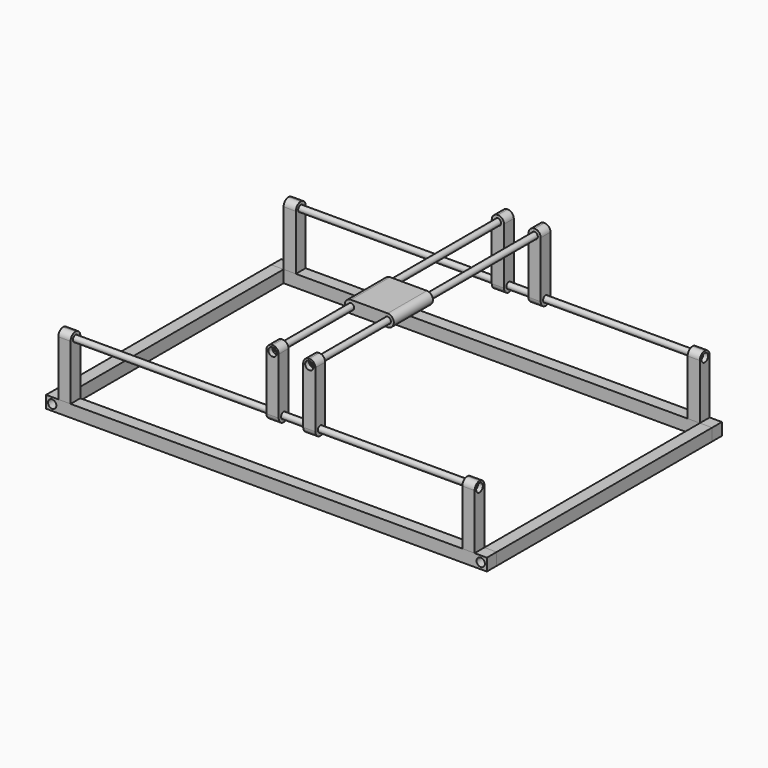
from build123d import *

# Parameters (mm, degrees)
F0_R                   = 2.159
F1_DEPTH               = 6.35
F0_W                   = 6.35
F0_H                   = 139.7
F2_DEPTH               = 6.35
F5_D                   = 2.54
F5_DEPTH               = 14.2875
F5_CBORE_D             = 4.318
F5_CBORE_DEPTH         = 6.35
F5_TIP                 = 0.7630929862
F5_2_D                 = 2.54
F5_2_DEPTH             = 14.2875
F5_2_CBORE_D           = 4.318
F5_2_CBORE_DEPTH       = 6.35
F5_2_TIP               = 0.7630929862
F5_3_D                 = 2.54
F5_3_DEPTH             = 14.2875
F5_3_CBORE_D           = 4.318
F5_3_CBORE_DEPTH       = 6.35
F5_3_TIP               = 0.7630929862
F5_ON_F3_D             = 2.54
F5_ON_F3_DEPTH         = 14.2875
F5_ON_F3_CBORE_D       = 4.318
F5_ON_F3_CBORE_DEPTH   = 6.35
F5_ON_F3_TIP           = 0.7630929862
F5_ON_F3_2_D           = 2.54
F5_ON_F3_2_DEPTH       = 14.2875
F5_ON_F3_2_CBORE_D     = 4.318
F5_ON_F3_2_CBORE_DEPTH = 6.35
F5_ON_F3_2_TIP         = 0.7630929862
F5_ON_F3_3_D           = 2.54
F5_ON_F3_3_DEPTH       = 14.2875
F5_ON_F3_3_CBORE_D     = 4.318
F5_ON_F3_3_CBORE_DEPTH = 6.35
F5_ON_F3_3_TIP         = 0.7630929862
F6_W                   = 6.35
F6_H                   = 6.35
F7_DEPTH               = 31.75
F8_R                   = 3.17499
F9_D                   = 2.5146
F9_DEPTH               = 15.2146
F9_CBORE_D             = 4.318
F9_CBORE_DEPTH         = 2.5146
F9_TIP                 = 0.7554620563
F9_2_D                 = 2.5146
F9_2_DEPTH             = 15.2146
F9_2_CBORE_D           = 4.318
F9_2_CBORE_DEPTH       = 2.5146
F9_2_TIP               = 0.7554620563
F9_3_D                 = 2.5146
F9_3_DEPTH             = 15.2146
F9_3_CBORE_D           = 4.318
F9_3_CBORE_DEPTH       = 2.5146
F9_3_TIP               = 0.7554620563
F10_R                  = 1.651
F11_DEPTH              = 1.27
F13_D                  = 2.5146
F13_CBORE_D            = 4.318
F13_CBORE_DEPTH        = 2.5146
F14_R                  = 1.5875
F15_DEPTH              = 102.87
F19_DEPTH              = 6.35
F21_DEPTH              = 6.35
F22_D                  = 2.5146
F22_CBORE_D            = 4.318
F22_CBORE_DEPTH        = 2.5146
F23_R                  = 1.6891
F23_R_2                = 1.2573
F24_DEPTH              = 1.27
F28_R                  = 1.5875
F29_DEPTH              = 71.12
F30_R                  = 1.651
F31_DEPTH              = 25.4


# Not quite as in the source:
# - a fillet or chamfer is up to 0.001 mm smaller than in the source, because OpenCascade refuses the exact size


with BuildPart() as f1:
    # F0 (on Top) → F1 (new body)
    with BuildSketch(Plane.XY):
        Polygon((-107.95, 69.85), (107.95, 69.85), (114.3, 69.85), (114.3, 76.2), (-114.3, 76.2), (-114.3, 69.85), align=None)
        with Locations((-104.775, 73.025)):
            Circle(F0_R, mode=Mode.SUBTRACT)
        with Locations((104.775, 73.025)):
            Circle(F0_R, mode=Mode.SUBTRACT)
        with Locations((-104.775, 73.025)):
            Circle(F0_R)
        with Locations((104.775, 73.025)):
            Circle(F0_R)
    extrude(amount=F1_DEPTH)

    # F5 on F3
    with Locations(Plane(origin=(0, 76.2, 0), x_dir=(-1, 0, 0), z_dir=(0, 1, 0))):
        with Locations((111.125, 3.175), (-111.125, 3.175)):
            CounterBoreHole(F5_ON_F3_D / 2, F5_ON_F3_CBORE_D / 2, F5_ON_F3_CBORE_DEPTH, depth=F5_ON_F3_DEPTH)
            with Locations((0, 0, -(F5_ON_F3_DEPTH + F5_ON_F3_TIP / 2))):  # 118° drill point
                Cone(0, F5_ON_F3_D / 2, F5_ON_F3_TIP, mode=Mode.SUBTRACT)

    # F9
    with Locations(Plane(origin=(0, 0, 0), x_dir=(1, 0, 0), z_dir=(0, 0, -1))):
        with Locations((-104.775, 73.025), (104.775, 73.025), (104.775, -73.025), (-104.775, -73.025)):
            CounterBoreHole(F9_D / 2, F9_CBORE_D / 2, F9_CBORE_DEPTH, depth=F9_DEPTH)
            with Locations((0, 0, -(F9_DEPTH + F9_TIP / 2))):  # 118° drill point
                Cone(0, F9_D / 2, F9_TIP, mode=Mode.SUBTRACT)


with BuildPart() as f1b:
    # F0 (on Top) → F1, piece 2 (new body)
    with BuildSketch(Plane.XY):
        Polygon((114.3, -69.85), (107.95, -69.85), (-107.95, -69.85), (-114.3, -69.85), (-114.3, -76.2), (114.3, -76.2), align=None)
        with Locations((-104.775, -73.025)):
            Circle(F0_R, mode=Mode.SUBTRACT)
        with Locations((104.775, -73.025)):
            Circle(F0_R, mode=Mode.SUBTRACT)
        with Locations((104.775, -73.025)):
            Circle(F0_R)
        with Locations((-104.775, -73.025)):
            Circle(F0_R)
    extrude(amount=F1_DEPTH)

    # F5
    with Locations(Plane.XZ.offset(76.2)):
        with Locations((111.125, 3.175), (-111.125, 3.175)):
            CounterBoreHole(F5_D / 2, F5_CBORE_D / 2, F5_CBORE_DEPTH, depth=F5_DEPTH)
            with Locations((0, 0, -(F5_DEPTH + F5_TIP / 2))):  # 118° drill point
                Cone(0, F5_D / 2, F5_TIP, mode=Mode.SUBTRACT)

    # F9#2
    with Locations(Plane(origin=(0, 0, 0), x_dir=(1, 0, 0), z_dir=(0, 0, -1))):
        with Locations((-104.775, 73.025), (104.775, 73.025), (104.775, -73.025), (-104.775, -73.025)):
            CounterBoreHole(F9_2_D / 2, F9_2_CBORE_D / 2, F9_2_CBORE_DEPTH, depth=F9_2_DEPTH)
            with Locations((0, 0, -(F9_2_DEPTH + F9_2_TIP / 2))):  # 118° drill point
                Cone(0, F9_2_D / 2, F9_2_TIP, mode=Mode.SUBTRACT)


with BuildPart() as f2:
    # F0 (on Top) → F2 (new body)
    with BuildSketch(Plane.XY):
        with Locations((-111.125, 0)):
            Rectangle(F0_W, F0_H)
    extrude(amount=F2_DEPTH)

    # F5#2
    with Locations(Plane.XZ.offset(76.2)):
        with Locations((111.125, 3.175), (-111.125, 3.175)):
            CounterBoreHole(F5_2_D / 2, F5_2_CBORE_D / 2, F5_2_CBORE_DEPTH, depth=F5_2_DEPTH)
            with Locations((0, 0, -(F5_2_DEPTH + F5_2_TIP / 2))):  # 118° drill point
                Cone(0, F5_2_D / 2, F5_2_TIP, mode=Mode.SUBTRACT)

    # F5 on F3#2
    with Locations(Plane(origin=(0, 76.2, 0), x_dir=(-1, 0, 0), z_dir=(0, 1, 0))):
        with Locations((111.125, 3.175), (-111.125, 3.175)):
            CounterBoreHole(F5_ON_F3_2_D / 2, F5_ON_F3_2_CBORE_D / 2, F5_ON_F3_2_CBORE_DEPTH, depth=F5_ON_F3_2_DEPTH)
            with Locations((0, 0, -(F5_ON_F3_2_DEPTH + F5_ON_F3_2_TIP / 2))):  # 118° drill point
                Cone(0, F5_ON_F3_2_D / 2, F5_ON_F3_2_TIP, mode=Mode.SUBTRACT)


with BuildPart() as f2b:
    # F0 (on Top) → F2, piece 2 (new body)
    with BuildSketch(Plane.XY):
        with Locations((111.125, 0)):
            Rectangle(F0_W, F0_H)
    extrude(amount=F2_DEPTH)

    # F5#3
    with Locations(Plane.XZ.offset(76.2)):
        with Locations((111.125, 3.175), (-111.125, 3.175)):
            CounterBoreHole(F5_3_D / 2, F5_3_CBORE_D / 2, F5_3_CBORE_DEPTH, depth=F5_3_DEPTH)
            with Locations((0, 0, -(F5_3_DEPTH + F5_3_TIP / 2))):  # 118° drill point
                Cone(0, F5_3_D / 2, F5_3_TIP, mode=Mode.SUBTRACT)

    # F5 on F3#3
    with Locations(Plane(origin=(0, 76.2, 0), x_dir=(-1, 0, 0), z_dir=(0, 1, 0))):
        with Locations((111.125, 3.175), (-111.125, 3.175)):
            CounterBoreHole(F5_ON_F3_3_D / 2, F5_ON_F3_3_CBORE_D / 2, F5_ON_F3_3_CBORE_DEPTH, depth=F5_ON_F3_3_DEPTH)
            with Locations((0, 0, -(F5_ON_F3_3_DEPTH + F5_ON_F3_3_TIP / 2))):  # 118° drill point
                Cone(0, F5_ON_F3_3_D / 2, F5_ON_F3_3_TIP, mode=Mode.SUBTRACT)


with BuildPart() as f7:
    # F6 (on face) → F7 (new body)
    with BuildSketch(Plane.XY.offset(6.35)):
        with Locations((-104.775, 73.025)):
            Rectangle(F6_W, F6_H)
    extrude(amount=F7_DEPTH)

    # F8 (radius 3.175 in the source; OpenCascade refuses exactly that, so slightly less here)
    f8_edges = [f7.edges().sort_by_distance(p)[0] for p in [
        (-104.775, 69.85, 38.1),
        (-104.775, 76.2, 38.1),
    ]]
    fillet(f8_edges, radius=F8_R)

    # F9#3
    with Locations(Plane(origin=(0, 0, 0), x_dir=(1, 0, 0), z_dir=(0, 0, -1))):
        with Locations((-104.775, 73.025), (104.775, 73.025), (104.775, -73.025), (-104.775, -73.025)):
            CounterBoreHole(F9_3_D / 2, F9_3_CBORE_D / 2, F9_3_CBORE_DEPTH, depth=F9_3_DEPTH)
            with Locations((0, 0, -(F9_3_DEPTH + F9_3_TIP / 2))):  # 118° drill point
                Cone(0, F9_3_D / 2, F9_3_TIP, mode=Mode.SUBTRACT)

    # F10 (on face) → F11 (cut)
    with BuildSketch(Plane.YZ.offset(-101.6)):
        with Locations((73.025, 34.925)):
            Circle(F10_R)
    extrude(amount=-F11_DEPTH, mode=Mode.SUBTRACT)

    # F13 (through all)
    with Locations(Plane(origin=(-107.95, 0, 0), x_dir=(0, -1, 0), z_dir=(-1, 0, 0))):
        with Locations((-73.025, 34.925)):
            CounterBoreHole(F13_D / 2, F13_CBORE_D / 2, F13_CBORE_DEPTH)


with BuildPart() as f15:
    # F14 (on Right) → F15 (new body, symmetric)
    with BuildSketch(Plane.YZ):
        with Locations((73.025, 34.925)):
            Circle(F14_R)
    extrude(amount=F15_DEPTH, both=True)


with BuildPart() as f16_1:
    # F16: instance of F7
    add(f7.part.mirror(Plane.YZ))


with BuildPart() as f17_1:
    # F17: instance of F16_1
    add(f16_1.part.mirror(Plane.XZ))


with BuildPart() as f17_2:
    # F17: instance of F7
    add(f7.part.mirror(Plane.XZ))


with BuildPart() as f17_3:
    # F17: instance of F15
    add(f15.part.mirror(Plane.XZ))


with BuildPart() as f19:
    # F18 (on Right) → F19 (new body)
    with BuildSketch(Plane.YZ):
        with BuildLine():
            ThreePointArc((76.2, 34.925), (75.2700640303, 37.1700640303), (73.025, 38.1))
            ThreePointArc((73.025, 38.1), (70.7799359697, 37.1700640303), (69.85, 34.925))
            ThreePointArc((69.85, 34.925), (73.025, 31.75), (76.2, 34.925))
        make_face()
        with BuildLine():
            ThreePointArc((73.025, 36.576), (74.1924332957, 36.0924332957), (74.676, 34.925))
            ThreePointArc((74.676, 34.925), (71.8575667043, 33.7575667043), (73.025, 36.576))
        make_face(mode=Mode.SUBTRACT)
        with BuildLine():
            ThreePointArc((69.85, 34.925), (70.7799359697, 37.1700640303), (73.025, 38.1))
            ThreePointArc((73.025, 38.1), (75.2700640303, 37.1700640303), (76.2, 34.925))
            Line((76.2, 34.925), (76.2, 67.31))
            Line((76.2, 67.31), (69.85, 67.31))
            Line((69.85, 67.31), (69.85, 34.925))
        make_face()
    extrude(amount=F19_DEPTH)

    # F20 (on face) → F21 (cut, through all)
    with BuildSketch(Plane(origin=(0, 76.2, 0), x_dir=(-1, 0, 0), z_dir=(0, 1, 0))):
        with BuildLine():
            ThreePointArc((-3.175, 67.31), (-0.9299359697, 66.3800640303), (0, 64.135))
            Line((0, 64.135), (0, 67.31))
            Line((0, 67.31), (-3.175, 67.31))
        make_face()
        with BuildLine():
            ThreePointArc((-6.35, 64.135), (-5.4200640303, 66.3800640303), (-3.175, 67.31))
            Line((-3.175, 67.31), (-6.35, 67.31))
            Line((-6.35, 67.31), (-6.35, 64.135))
        make_face()
    extrude(amount=-F21_DEPTH, mode=Mode.SUBTRACT)

    # F22 (through all)
    with Locations(Plane(origin=(0, 76.2, 0), x_dir=(-1, 0, 0), z_dir=(0, 1, 0))):
        with Locations((-3.175, 64.135)):
            CounterBoreHole(F22_D / 2, F22_CBORE_D / 2, F22_CBORE_DEPTH)

    # F23 (on face) → F24 (cut)
    with BuildSketch(Plane.XZ.offset(-69.85)):
        with Locations((3.175, 64.135)):
            Circle(F23_R)
        with Locations((3.175, 64.135)):
            Circle(F23_R_2, mode=Mode.SUBTRACT)
    extrude(amount=-F24_DEPTH, mode=Mode.SUBTRACT)


with BuildPart() as f26_1:
    # F26: instance of F19
    add(f19.part.mirror(Plane.YZ.offset(12.7)))


with BuildPart() as f27_1:
    # F27: instance of F26_1
    add(f26_1.part.mirror(Plane.XZ))


with BuildPart() as f27_2:
    # F27: instance of F19
    add(f19.part.mirror(Plane.XZ))


with BuildPart() as f29:
    # F28 (on Front) → F29 (new body, symmetric)
    with BuildSketch(Plane.XZ):
        with Locations((22.225, 64.135)):
            Circle(F28_R)
    extrude(amount=F29_DEPTH, both=True)


with BuildPart() as f29b:
    # F28 (on Front) → F29, piece 2 (new body, symmetric)
    with BuildSketch(Plane.XZ):
        with Locations((3.175, 64.135)):
            Circle(F28_R)
    extrude(amount=F29_DEPTH, both=True)


with BuildPart() as f31:
    # F30 (on Front) → F31 (new body)
    with BuildSketch(Plane.XZ):
        with BuildLine():
            Line((22.225, 67.31), (3.175, 67.31))
            ThreePointArc((3.175, 67.31), (0, 64.135), (3.175, 60.96))
            Line((3.175, 60.96), (22.225, 60.96))
            ThreePointArc((22.225, 60.96), (25.4, 64.135), (22.225, 67.31))
        make_face()
        with Locations((3.175, 64.135)):
            Circle(F30_R, mode=Mode.SUBTRACT)
        with Locations((22.225, 64.135)):
            Circle(F30_R, mode=Mode.SUBTRACT)
    extrude(amount=F31_DEPTH)


solid = Compound([f1.part, f1b.part, f2.part, f2b.part, f7.part, f15.part, f16_1.part, f17_1.part, f17_2.part, f17_3.part, f19.part, f26_1.part, f27_1.part, f27_2.part, f29.part, f29b.part, f31.part])
